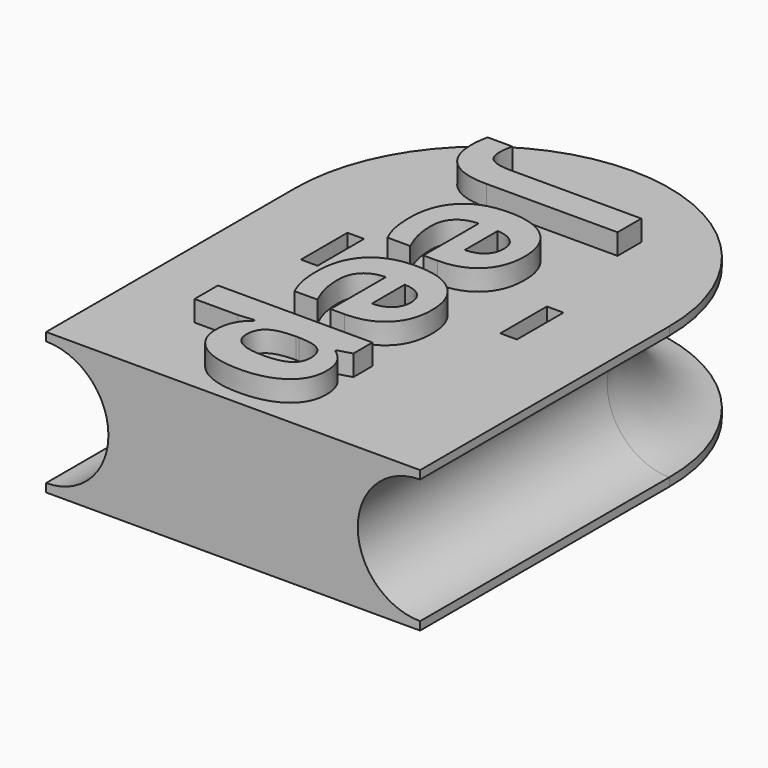
from build123d import *

# Parameters (mm, degrees)
F1_DEPTH     = 21.59
F2_R         = 9.525
F4_TEXT_SIZE = 30.0205382592
F5_DEPTH     = 3.175
F6_W         = 2.54
F6_H         = 8.89
F7_DEPTH     = 25.4


# Not quite as in the source:
# - Text() gives the source's letters only with a copy of the font that has no kerning and outlines rounded to 1/6400 em; it was checked with that copy


with BuildPart() as f1:
    # F0 (on Top) → F1 (new body)
    with BuildSketch(Plane.XY):
        with BuildLine():
            Line((0, 47.625), (0, 0))
            Line((0, 0), (57.15, 0))
            Line((57.15, 0), (57.15, 47.625))
            ThreePointArc((57.15, 47.625), (28.575, 76.2), (0, 47.625))
        make_face()
    extrude(amount=F1_DEPTH)

    # F3: sweep along a path in F3_path
    with BuildLine(Plane(origin=(0, 47.625, 21.59), x_dir=(0, 1, 0), z_dir=(0, 0, 1))) as f3_path:
        Line((-47.625, 0), (0, 0))
        ThreePointArc((0, 0), (28.575, -28.575), (0, -57.15))
        Line((0, -57.15), (-47.625, -57.15))
    # F2 (on Front) → F3 (sweep, cut)
    with BuildSketch(Plane.XZ):
        with Locations((0, 10.795)):
            Circle(F2_R)
    sweep(path=f3_path.line, mode=Mode.SUBTRACT)

    # F4 (on face) → F5 (join)
    with BuildSketch(Plane.XY.offset(21.59)):
        with Locations(Location((19.5315051824, 65.1846472174), (0, 0, -90))):
            Text('Jeep', F4_TEXT_SIZE, font='Open Sans', font_style=FontStyle.BOLD, text_align=(TextAlign.LEFT, TextAlign.BOTTOM))
    extrude(amount=F5_DEPTH)

    # F6 (on face) → F7 (cut)
    with BuildSketch(Plane.XY.offset(21.59)):
        with Locations((13.335, 38.0319244497)):
            Rectangle(F6_W, F6_H)
        with Locations((43.815, 38.0238)):
            Rectangle(F6_W, F6_H)
    extrude(amount=-F7_DEPTH, mode=Mode.SUBTRACT)


solid = f1.part
